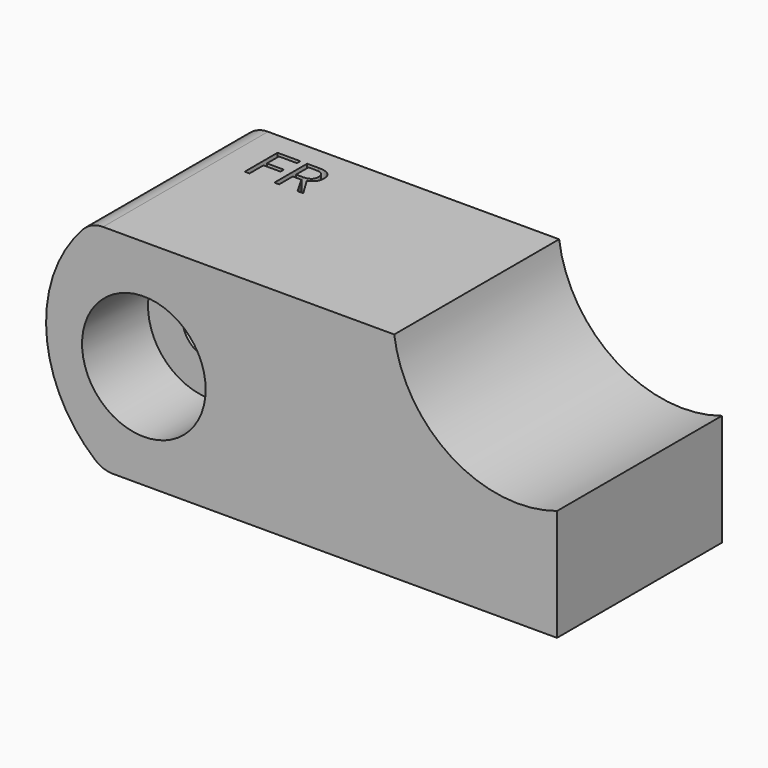
from build123d import *

# Parameters (mm, degrees)
F1_DEPTH     = 47.625
F2_R         = 6.35
F3_R         = 14.2780224538
F4_DEPTH     = 47.626
F5_TEXT_SIZE = 13.2534400715
F6_DEPTH     = 6.35
F7_R         = 14.2780224538
F7_R_2       = 6.35
F8_DEPTH     = 28.575


# Not quite as in the source:
# - Text() gives the source's letters only with a copy of the font that has no kerning and outlines rounded to 1/6400 em; it was checked with that copy


with BuildPart() as f1:
    # F0 (on Front) → F1 (new body)
    with BuildSketch(Plane.XZ):
        with BuildLine():
            Line((21.3502769062, 28.2528719176), (-48.4997230938, 28.2528719176))
            ThreePointArc((-48.4997230938, 28.2528719176), (-59.0377618998, 2.8678235631), (-45.8169638626, -21.2290941049))
            Line((-45.8169638626, -21.2290941049), (58.9580361374, -21.2290941049))
            Line((58.9580361374, -21.2290941049), (58.9580361374, 4.5773058951))
            ThreePointArc((58.9580361374, 4.5773058951), (34.5972835683, 7.5882021525), (21.3502769062, 28.2528719176))
        make_face()
    extrude(amount=F1_DEPTH)

    # F2
    f2_edges = [f1.edges().sort_by_distance(p)[0] for p in [
        (-48.499723, -23.8125, 28.252872),
        (-45.816964, -23.8125, -21.229094),
    ]]
    fillet(f2_edges, radius=F2_R)

    # F3 (on face) → F4 (cut, through all)
    with BuildSketch(Plane.XZ.offset(47.625)):
        with Locations((-36.4931114018, 2.9011261649)):
            Circle(F3_R)
    extrude(amount=-F4_DEPTH, mode=Mode.SUBTRACT)

    # F5 (on face) → F6 (cut)
    with BuildSketch(Plane.XY.offset(28.2528719176)):
        with Locations((-40.7390370965, -14.803073369)):
            Text('FR', F5_TEXT_SIZE, font='Open Sans', text_align=(TextAlign.LEFT, TextAlign.BOTTOM))
    extrude(amount=-F6_DEPTH, mode=Mode.SUBTRACT)

    # F7 (on Front) → F8 (join)
    with BuildSketch(Plane.XZ):
        with Locations((-36.4931114018, 2.9011261649)):
            Circle(F7_R)
        with Locations((-36.4931114018, 2.9011261649)):
            Circle(F7_R_2, mode=Mode.SUBTRACT)
    extrude(amount=F8_DEPTH)


solid = f1.part
